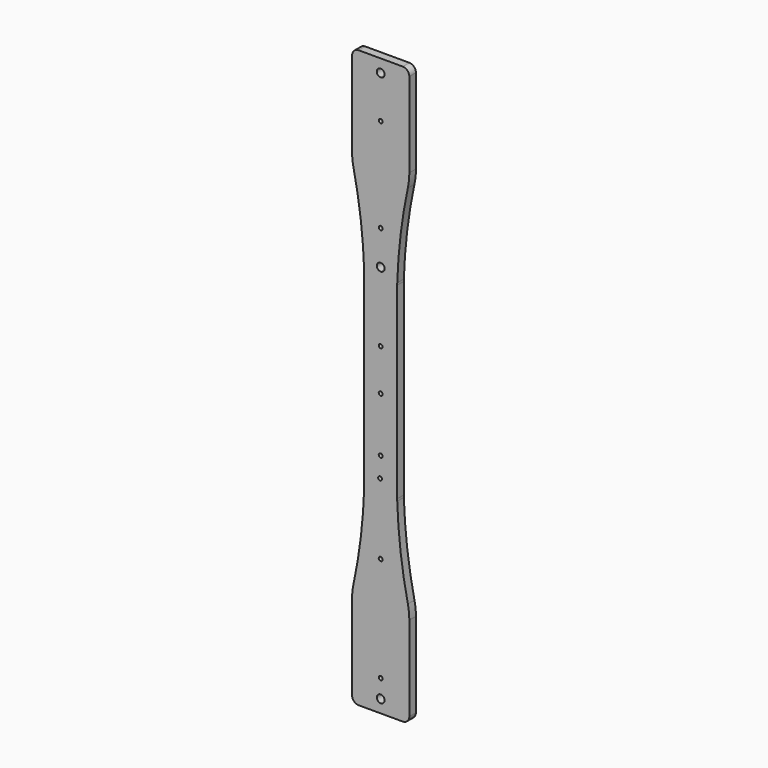
from build123d import *

# Parameters (mm, degrees)
F0_R        = 1.5
F0_R_2      = 3
F1_DEPTH    = 6.35
F2_R        = 5.08
F3_T1_DEPTH = 6.35
F3_T3_DEPTH = 34.0624500619


# Not quite as in the source:
# - a fillet or chamfer that OpenCascade refuses, or shapes differently, is made with other operations: its cross-section is extruded or revolved along the edge and cut away or added
# - a feature names something its author has since deleted; it is built from what else it names


with BuildPart() as f1:
    # F0 (on Front) → F1 (new body)
    with BuildSketch(Plane.XZ):
        with BuildLine():
            Line((-22, -189.9611499309), (-4.6853246795, -189.9611499309))
            Line((-4.6853246795, -189.9611499309), (0, -189.9611499309))
            Line((0, -189.9611499309), (4.6853246795, -189.9611499309))
            Line((4.6853246795, -189.9611499309), (22, -189.9611499309))
            Line((22, -189.9611499309), (22, -172.8709284505))
            Line((22, -172.8709284505), (22, -161.9910197589))
            Line((22, -161.9910197589), (22, -114.1058849427))
            ThreePointArc((22, -114.1058849427), (15.5787747464, -77.9579307824), (12.7, -41.3571195934))
            Line((12.7, -41.3571195934), (12.7, 104.7939062119))
            ThreePointArc((12.7, 104.7939062119), (15.5787747464, 141.3947174009), (22, 177.5426715612))
            Line((22, 177.5426715612), (22, 225.4278063774))
            Line((22, 225.4278063774), (22, 236.307715069))
            Line((22, 236.307715069), (22, 253.3979365494))
            Line((22, 253.3979365494), (4.6853246795, 253.3979365494))
            Line((4.6853246795, 253.3979365494), (0, 253.3979365494))
            Line((0, 253.3979365494), (-4.6853246795, 253.3979365494))
            Line((-4.6853246795, 253.3979365494), (-22, 253.3979365494))
            Line((-22, 253.3979365494), (-22, 236.307715069))
            Line((-22, 236.307715069), (-22, 225.4278063774))
            Line((-22, 225.4278063774), (-22, 177.5426715612))
            ThreePointArc((-22, 177.5426715612), (-15.5787747464, 141.3947174009), (-12.7, 104.7939062119))
            Line((-12.7, 104.7939062119), (-12.7, -41.3571195934))
            ThreePointArc((-12.7, -41.3571195934), (-15.5787747464, -77.9579307824), (-22, -114.1058849427))
            Line((-22, -114.1058849427), (-22, -161.9910197589))
            Line((-22, -161.9910197589), (-22, -172.8709284505))
            Line((-22, -172.8709284505), (-22, -189.9611499309))
        make_face()
        with Locations((-0.4384766798, -31.0452261312)):
            Circle(F0_R, mode=Mode.SUBTRACT)
        with Locations((0, -180.0831407309)):
            Circle(F0_R_2, mode=Mode.SUBTRACT)
        with Locations((0, -166.0831407309)):
            Circle(F0_R, mode=Mode.SUBTRACT)
        with Locations((0, -85.4520261312)):
            Circle(F0_R, mode=Mode.SUBTRACT)
        with Locations((0, -15.4520261312)):
            Circle(F0_R, mode=Mode.SUBTRACT)
        with Locations((0, 26.5547856688)):
            Circle(F0_R, mode=Mode.SUBTRACT)
        with BuildLine():
            ThreePointArc((1.5, 58.5587856688), (-1.0606601718, 57.4981254971), (0, 60.0587856688))
            ThreePointArc((0, 60.0587856688), (1.0606601718, 59.6194458406), (1.5, 58.5587856688))
        make_face(mode=Mode.SUBTRACT)
        with BuildLine():
            ThreePointArc((0, 109.0876222849), (-3, 112.0876222849), (0, 115.0876222849))
            ThreePointArc((0, 115.0876222849), (2.1213203436, 114.2089426284), (3, 112.0876222849))
            ThreePointArc((3, 112.0876222849), (2.1213203436, 109.9663019413), (0, 109.0876222849))
        make_face(mode=Mode.SUBTRACT)
        with BuildLine():
            ThreePointArc((0, 137.0615974688), (-1.5, 138.5615974688), (0, 140.0615974688))
            ThreePointArc((0, 140.0615974688), (1.0606601718, 139.6222576406), (1.5, 138.5615974688))
            ThreePointArc((1.5, 138.5615974688), (1.0606601718, 137.5009372971), (0, 137.0615974688))
        make_face(mode=Mode.SUBTRACT)
        with BuildLine():
            ThreePointArc((0, 209.4587856688), (-1.5, 210.9587856688), (0, 212.4587856688))
            ThreePointArc((0, 212.4587856688), (1.0606601718, 212.0194458406), (1.5, 210.9587856688))
            ThreePointArc((1.5, 210.9587856688), (1.0606601718, 209.8981254971), (0, 209.4587856688))
        make_face(mode=Mode.SUBTRACT)
        with BuildLine():
            ThreePointArc((0, 240.5199192026), (-3, 243.5199192026), (0, 246.5199192026))
            ThreePointArc((0, 246.5199192026), (2.1213203436, 245.6412395461), (3, 243.5199192026))
            ThreePointArc((3, 243.5199192026), (2.1213203436, 241.398598859), (0, 240.5199192026))
        make_face(mode=Mode.SUBTRACT)
    extrude(amount=F1_DEPTH)

    # F2
    f2_edges = [f1.edges().sort_by_distance(p)[0] for p in [
        (-22, -3.175, 253.397937),
        (22, -3.175, 253.397937),
        (22, -3.175, -189.96115),
        (-22, -3.175, -189.96115),
    ]]
    fillet(f2_edges, radius=F2_R)

    # F3: fillet of radius 50.8 on 8 edges, made by hand

    # F3_s2 → F3_t1 (join)
    with BuildSketch(Plane.XZ):
        with BuildLine():
            ThreePointArc((-12.7, 104.0086355302), (-12.7065317021, 104.8232386677), (-12.7261251288, 105.6376323271))
            ThreePointArc((-12.7261251288, 105.6376323271), (-12.7128266876, 105.2157765732), (-12.7, 104.7939062119))
            Line((-12.7, 104.7939062119), (-12.7, 104.0086355302))
        make_face()
        with BuildLine():
            ThreePointArc((12.7, 104.0086355302), (12.7065317021, 104.8232386677), (12.7261251288, 105.6376323271))
            ThreePointArc((12.7261251288, 105.6376323271), (12.7128266876, 105.2157765732), (12.7, 104.7939062119))
            Line((12.7, 104.7939062119), (12.7, 104.0086355302))
        make_face()
        with BuildLine():
            ThreePointArc((12.7261251288, -42.2008457086), (12.7065317021, -41.3864520492), (12.7, -40.5718489117))
            Line((12.7, -40.5718489117), (12.7, -41.3571195934))
            ThreePointArc((12.7, -41.3571195934), (12.7128266876, -41.7789899547), (12.7261251288, -42.2008457086))
        make_face()
        with BuildLine():
            ThreePointArc((-12.7261251288, -42.2008457086), (-12.7065317021, -41.3864520492), (-12.7, -40.5718489116))
            Line((-12.7, -40.5718489116), (-12.7, -41.3571195934))
            ThreePointArc((-12.7, -41.3571195934), (-12.7128266876, -41.7789899547), (-12.7261251288, -42.2008457086))
        make_face()
    extrude(amount=F3_T1_DEPTH)

    # F3_s4 → F3_t3 (cut)
    with BuildSketch(Plane.XZ.offset(-13.856225031)):
        with BuildLine():
            ThreePointArc((-22, -119.6483749551), (-21.7184280188, -114.3071737314), (-20.8768334444, -109.025182453))
            ThreePointArc((-20.8768334444, -109.025182453), (-21.429661091, -111.5674692633), (-22, -114.1058849427))
            Line((-22, -114.1058849427), (-22, -119.6483749551))
        make_face()
        with BuildLine():
            ThreePointArc((22, -119.6483749551), (21.7184280188, -114.3071737314), (20.8768334444, -109.025182453))
            ThreePointArc((20.8768334444, -109.025182453), (21.429661091, -111.5674692633), (22, -114.1058849427))
            Line((22, -114.1058849427), (22, -119.6483749551))
        make_face()
        with BuildLine():
            ThreePointArc((20.8768334444, 172.4619690715), (21.7184280188, 177.7439603499), (22, 183.0851615736))
            Line((22, 183.0851615736), (22, 177.5426715612))
            ThreePointArc((22, 177.5426715612), (21.429661091, 175.0042558818), (20.8768334444, 172.4619690715))
        make_face()
        with BuildLine():
            ThreePointArc((-20.8768334444, 172.4619690715), (-21.7184280188, 177.7439603499), (-22, 183.0851615736))
            Line((-22, 183.0851615736), (-22, 177.5426715612))
            ThreePointArc((-22, 177.5426715612), (-21.429661091, 175.0042558818), (-20.8768334444, 172.4619690715))
        make_face()
    extrude(amount=F3_T3_DEPTH, mode=Mode.SUBTRACT)


solid = f1.part
